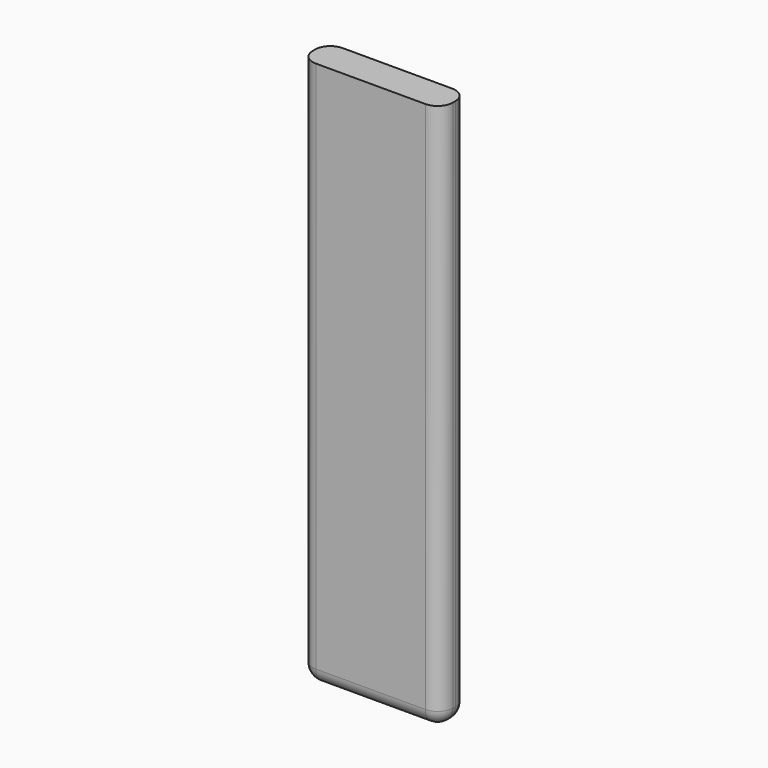
from build123d import *

# Parameters (mm, degrees)
F0_W         = 46
F0_H         = 11
F1_DEPTH     = 180
F2_T         = -2.5
F3_T1_DEPTH  = 71
F4_R         = 5
F5_T1_DEPTH  = 187.5
F5_T3_DEPTH  = 1
F5_T6_ANGLE  = 90
F5_T8_ANGLE  = 89.9999999974
F5_T10_ANGLE = 90
F5_T12_ANGLE = 89.9999999974


# Not quite as in the source:
# - a fillet or chamfer that OpenCascade refuses, or shapes differently, is made with other operations: its cross-section is extruded or revolved along the edge and cut away or added


with BuildPart() as f1:
    # F0 (on Top) → F1 (new body)
    with BuildSketch(Plane.XY):
        with Locations((23, -5.5)):
            Rectangle(F0_W, F0_H)
    extrude(amount=F1_DEPTH)

    # F2
    f2_openings = [f1.faces().sort_by_distance(p)[0] for p in [
        (23, 0, 90),
    ]]
    offset(amount=F2_T, openings=f2_openings)

    # F3: fillet of radius 5 on 1 edges, made by hand

    # F3_s2 → F3_t1 (cut)
    with BuildSketch(Plane.YZ.offset(-12.5)):
        with BuildLine():
            ThreePointArc((-5, 0), (-1.4644660941, 1.4644660941), (0, 5))
            Line((0, 5), (0, 0))
            Line((0, 0), (-5, 0))
        make_face()
    extrude(amount=F3_T1_DEPTH, mode=Mode.SUBTRACT)

    # F4
    f4_edges = [f1.edges().sort_by_distance(p)[0] for p in [
        (23, -11, 0),
    ]]
    fillet(f4_edges, radius=F4_R)

    # F5: fillet of radius 5 on 2 edges, made by hand

    # F5_s2 → F5_t1 (cut)
    with BuildSketch(Plane.XY.offset(5)):
        with BuildLine():
            ThreePointArc((0, -6), (1.4644660941, -9.5355339059), (5, -11))
            Line((5, -11), (0, -11))
            Line((0, -11), (0, -6))
        make_face()
        with BuildLine():
            ThreePointArc((41, -11), (44.5355339059, -9.5355339059), (46, -6))
            Line((46, -6), (46, -11))
            Line((46, -11), (41, -11))
        make_face()
        with BuildLine():
            ThreePointArc((41, 0), (44.5355339059, -1.4644660941), (46, -5))
            Line((46, -5), (46, 0))
            Line((46, 0), (41, 0))
        make_face()
        with BuildLine():
            ThreePointArc((0, -5), (1.4644660941, -1.4644660941), (5, 0))
            Line((5, 0), (0, 0))
            Line((0, 0), (0, -5))
        make_face()
    extrude(amount=F5_T1_DEPTH, mode=Mode.SUBTRACT)

    # F5_s4 → F5_t3 (cut)
    with BuildSketch(Plane.XZ.offset(5)):
        with BuildLine():
            ThreePointArc((41, 0), (44.5355339059, 1.4644660941), (46, 5))
            Line((46, 5), (46, 0))
            Line((46, 0), (41, 0))
        make_face()
        with BuildLine():
            ThreePointArc((0, 5), (1.4644660941, 1.4644660941), (5, 0))
            Line((5, 0), (0, 0))
            Line((0, 0), (0, 5))
        make_face()
    extrude(amount=F5_T3_DEPTH, mode=Mode.SUBTRACT)

    # F5_s5 → F5_t6 (revolve, cut)
    with BuildSketch(Plane.XZ.offset(6)):
        with BuildLine():
            ThreePointArc((41, 0), (44.5355339059, 1.4644660941), (46, 5))
            Line((46, 5), (46, 0))
            Line((46, 0), (41, 0))
        make_face()
    revolve(axis=Axis((46, -6, 5), (-1, 0, 0)), revolution_arc=F5_T6_ANGLE, mode=Mode.SUBTRACT)

    # F5_s7 → F5_t8 (revolve, cut)
    with BuildSketch(Plane.XY.offset(5.0000000001)):
        with BuildLine():
            ThreePointArc((41, 0), (44.5355339059, -1.4644660941), (46, -5))
            Line((46, -5), (46, 0))
            Line((46, 0), (41, 0))
        make_face()
    revolve(axis=Axis((46, -5.0000000001, 5.0000000001), (-1, 0, 0)), revolution_arc=F5_T8_ANGLE, mode=Mode.SUBTRACT)

    # F5_s9 → F5_t10 (revolve, cut)
    with BuildSketch(Plane.XZ.offset(6)):
        with BuildLine():
            ThreePointArc((0, 5), (1.4644660941, 1.4644660941), (5, 0))
            Line((5, 0), (0, 0))
            Line((0, 0), (0, 5))
        make_face()
    revolve(axis=Axis((0, -6, 5), (-1, 0, 0)), revolution_arc=F5_T10_ANGLE, mode=Mode.SUBTRACT)

    # F5_s11 → F5_t12 (revolve, cut)
    with BuildSketch(Plane.XY.offset(5.0000000001)):
        with BuildLine():
            ThreePointArc((0, -5), (1.4644660941, -1.4644660941), (5, 0))
            Line((5, 0), (0, 0))
            Line((0, 0), (0, -5))
        make_face()
    revolve(axis=Axis((0, -5.0000000001, 5.0000000001), (-1, 0, 0)), revolution_arc=F5_T12_ANGLE, mode=Mode.SUBTRACT)


solid = f1.part
